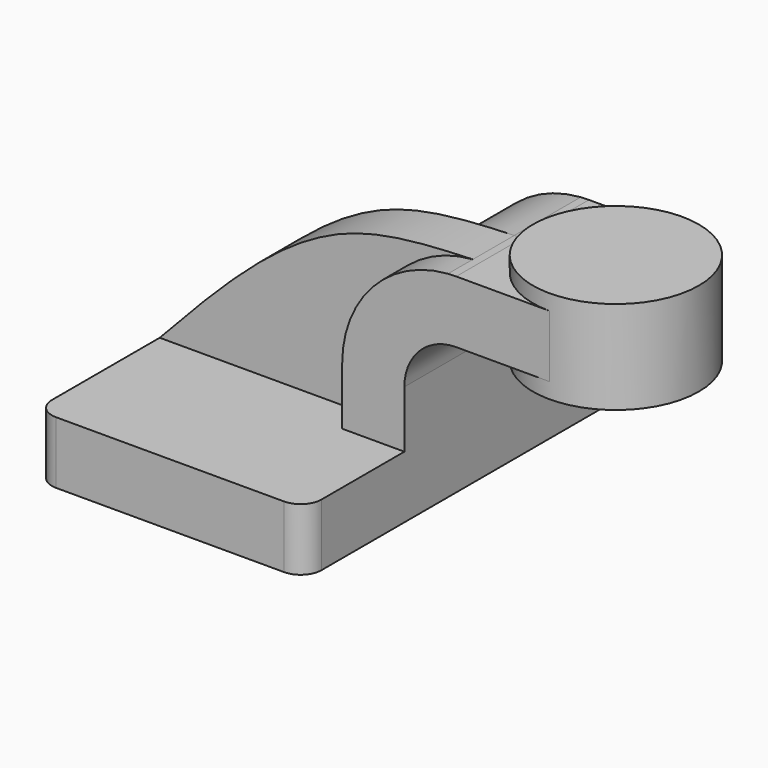
from build123d import *

# Parameters (mm, degrees)
F1_DEPTH = 63.5
F0_W     = 25.4
F0_H     = 19.05
F2_DEPTH = 25.4
F3_DEPTH = 15.875
F5_R     = 6.35


# Not quite as in the source:
# - a feature names something its author has since deleted; it is built from what else it names


with BuildPart() as f1:
    # F0 (on Front) → F1 (new body, symmetric)
    with BuildSketch(Plane.XZ):
        Polygon((41.275, -9.525), (41.275, 9.525), (22.225, 9.525), (-41.275, 9.525), (-41.275, -9.525), align=None)
    extrude(amount=F1_DEPTH, both=True)

    # F0 (on Front) → F2 (join, symmetric)
    with BuildSketch(Plane.XZ):
        with BuildLine():
            Line((22.225, 9.525), (41.275, 9.525))
            Line((41.275, 9.525), (41.275, 27.0002))
            ThreePointArc((41.275, 27.0002), (45.9246798487, 38.2255201513), (57.15, 42.8752))
            Line((57.15, 42.8752), (60.325, 42.8752))
            Line((60.325, 42.8752), (60.325, 61.9252))
            Line((60.325, 61.9252), (57.15, 61.9252))
            add(Edge.make_bspline(
                [(54.6259105013, 61.8338704526), (55.4670032291, 61.8648637063), (56.3085016145, 61.8950318532), (57.15, 61.9252)],
                knots=[0.9787843068, 0.9787843068, 0.9787843068, 0.9787843068, 1, 1, 1, 1], degree=3))
            ThreePointArc((54.6259105013, 61.8338704526), (31.5774614993, 50.7867697323), (22.225, 27.0002))
            Line((22.225, 27.0002), (22.225, 9.525))
        make_face()
        with Locations((73.025, 52.4002)):
            Rectangle(F0_W, F0_H)
    extrude(amount=F2_DEPTH, both=True)

    # F0 (on Front) → F3 (join)
    with BuildSketch(Plane.XZ):
        with BuildLine():
            Line((-41.275, 9.525), (22.225, 9.525))
            Line((22.225, 9.525), (22.225, 27.0002))
            ThreePointArc((22.225, 27.0002), (31.5774614993, 50.7867697323), (54.6259105013, 61.8338704526))
            add(Edge.make_bspline(
                [(-41.275, 9.525), (-31.2937791868, 20.1864348925), (-12.273821172, 40.5025913853), (17.5953077761, 60.105451895), (42.3186244489, 61.380361789), (54.6259105013, 61.8338704526)],
                knots=[0, 0, 0, 0, 0.3507319306, 0.6683457584, 0.9787843068, 0.9787843068, 0.9787843068, 0.9787843068], degree=3))
        make_face()
    extrude(amount=F3_DEPTH)

    # F0 (on Front) → F4 (revolve)
    with BuildSketch(Plane.XZ):
        Polygon((85.725, 61.9252), (85.725, 42.8752), (85.725, 38.1), (111.125, 38.1), (111.125, 66.675), (85.725, 66.675), align=None)
    revolve(axis=Axis((85.725, 0, 52.3875), (0, 0, -1)))

    # F5
    f5_edges = [f1.edges().sort_by_distance(p)[0] for p in [
        (-41.275, -63.5, 0),
        (-41.275, 63.5, 0),
        (41.275, 63.5, 0),
        (41.275, -63.5, 0),
    ]]
    fillet(f5_edges, radius=F5_R)


solid = f1.part
